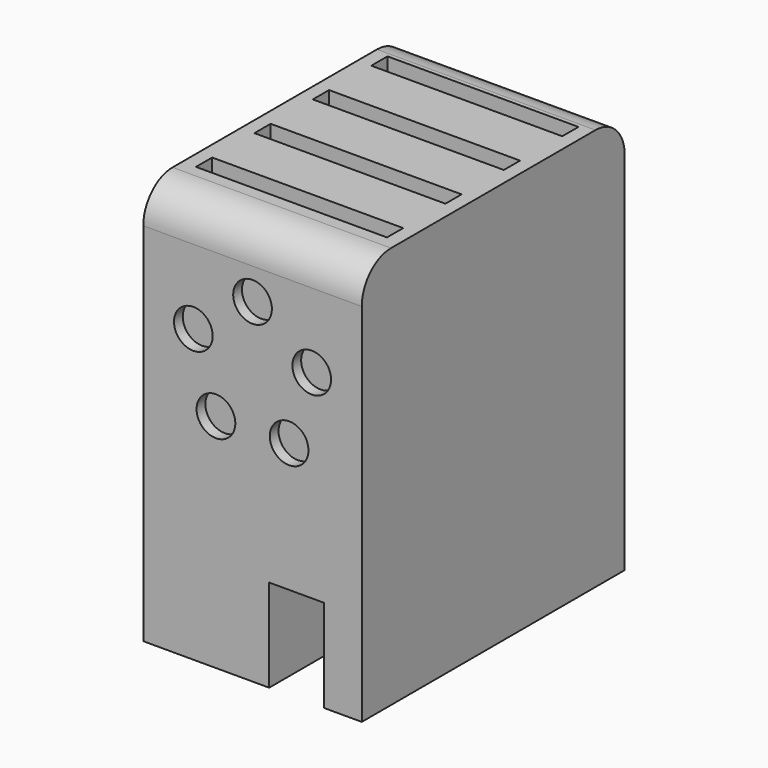
from build123d import *

# Parameters (mm, degrees)
F1_DEPTH  = 22.5
F3_W      = 26.150945574
F3_H      = 2.773584798
F4_DEPTH  = 18
F7_R      = 5
F6_W      = 35.4622639716
F6_H      = 18.6226405203
F8_DEPTH  = 1.5
F10_R     = 2.7697383404
F11_DEPTH = 1.5
F14_R     = 2.5
F15_DEPTH = 1.3
F17_R     = 2.6497529256
F18_DEPTH = 1.5


# Not quite as in the source:
# - a pattern or mirror of a feature is missing from the dataset's text; its kind, count and spacing are read off the source's solid


with BuildPart() as f1:
    # F0 (on Front) → F1 (new body, symmetric)
    with BuildSketch(Plane.XZ):
        Polygon((9.8066031933, -27.5377351791), (14.9575471878, -27.5377351791), (14.9575471878, 27.5377351791), (-14.9575471878, 27.5377351791), (-14.9575471878, -27.5377351791), (2.2783020977, -27.5377351791), (2.2783020977, -14.8584917188), (9.8066031933, -14.8584917188), align=None)
    extrude(amount=F1_DEPTH, both=True)

    # F3 (on offset) → F4 (cut)
    with BuildSketch(Plane.XY.offset(27.5377351791)):
        with Locations((0, 15.5518874526)):
            Rectangle(F3_W, F3_H)
        with Locations((0, 5.5518874526)):
            Rectangle(F3_W, F3_H)
        with Locations((0, -4.4481125474)):
            Rectangle(F3_W, F3_H)
        with Locations((0, -14.4481125474)):
            Rectangle(F3_W, F3_H)
    extrude(amount=-F4_DEPTH, mode=Mode.SUBTRACT)

    # F7
    f7_edges = [f1.edges().sort_by_distance(p)[0] for p in [
        (0, -22.5, 27.537735),
        (0, 22.5, 27.537735),
    ]]
    fillet(f7_edges, radius=F7_R)

    # F6 (on offset) → F8 (cut)
    with BuildSketch(Plane(origin=(-14.9575471878, 0, 0), x_dir=(0, -1, 0), z_dir=(-1, 0, 0))):
        with Locations((0, 14.6603807807)):
            Rectangle(F6_W, F6_H)
    extrude(amount=-F8_DEPTH, mode=Mode.SUBTRACT)

    # F10 (on offset) → F11 (join)
    with BuildSketch(Plane(origin=(-13.4575471878, 0, 0), x_dir=(0, -1, 0), z_dir=(-1, 0, 0))):
        with Locations((-8.6189499125, 18.3801390231)):
            Circle(F10_R)
        with Locations((8.6189499125, 18.3801390231)):
            Circle(F10_R)
        with BuildLine():
            Line((3.3579913629, 12.3015097342), (-3.90234219, 12.3015097342))
            ThreePointArc((-3.90234219, 12.3015097342), (-0.2721754136, 8.6713429578), (3.3579913629, 12.3015097342))
        make_face()
    extrude(amount=F11_DEPTH)

    # F13 (on offset) + F14 (on offset) → F15 (join)
    with BuildSketch(Plane(origin=(-14.9575471878, 0, 0), x_dir=(0, -1, 0), z_dir=(-1, 0, 0))):
        Polygon((-12.6108881086, -15.9375003353), (-7.5907266326, -15.9375003353), (-7.5907266326, -10.8266131394), (-2.5705651566, -10.8266131394), (-2.5705651566, -5.7157259434), (-7.5907266326, -5.7157259434), (-7.5907266326, -0.9375003353), (-12.6108881086, -0.9375003353), (-12.6108881086, -5.7157259434), (-17.5705651566, -5.7157259434), (-17.5705651566, -10.8266131394), (-12.6108881086, -10.8266131394), align=None)
    with BuildSketch(Plane(origin=(-14.9575471878, 0, 0), x_dir=(0, -1, 0), z_dir=(-1, 0, 0))):
        with Locations((10.3680184111, -5.60903208)):
            Circle(F14_R)
        with Locations((4.8680184111, -15.1353115216)):
            Circle(F14_R)
        with Locations((15.8680184111, -15.1353115216)):
            Circle(F14_R)
    extrude(amount=F15_DEPTH)

    # F17 (on offset) → F18 (cut)
    with BuildSketch(Plane(origin=(0, 22.5, 0), x_dir=(-1, 0, 0), z_dir=(0, 1, 0))):
        with Locations((0, 18.2300075523)):
            Circle(F17_R)
        with Locations((8.105232894, 12.3412111554)):
            Circle(F17_R)
        with Locations((5.0093094152, 2.8129384324)):
            Circle(F17_R)
        with Locations((-5.0093094152, 2.8129384324)):
            Circle(F17_R)
        with Locations((-8.105232894, 12.3412111554)):
            Circle(F17_R)
    f18 = extrude(amount=-F18_DEPTH, mode=Mode.SUBTRACT)

    # F18_copies: F18 across plane
    add(f18.mirror(Plane(origin=(0, 0, 0), x_dir=(0, 0, -1), z_dir=(0, -1, 0))), mode=Mode.SUBTRACT)


solid = f1.part
